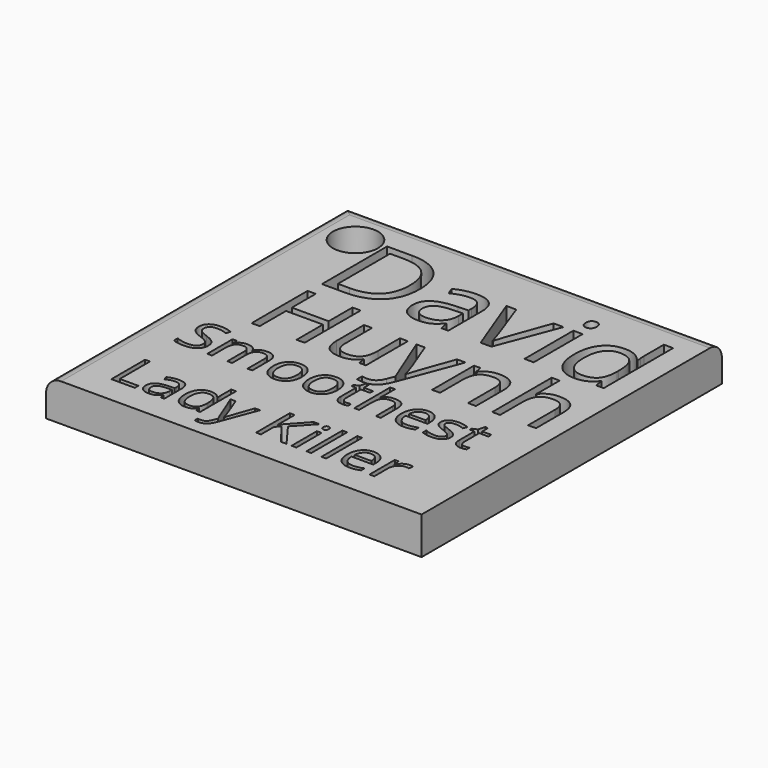
from build123d import *

# Parameters (mm, degrees)
F0_W         = 50
F0_H         = 50
F0_R         = 3
F1_DEPTH     = 5
F2_TEXT_SIZE = 13.0405990525
F4_DEPTH     = 5.001
F5_R         = 2
F6_TEXT_SIZE = 15.2046088971
F7_DEPTH     = 5.0010001
F3_TEXT_SIZE = 7.860235193
F8_DEPTH     = 5.0010001


# Not quite as in the source:
# - Text() gives the source's letters only with a copy of the font that has no kerning and outlines rounded to 1/6400 em; it was checked with that copy


with BuildPart() as f1:
    # F0 (on Top) → F1 (new body)
    with BuildSketch(Plane.XY):
        with Locations((25, -25)):
            Rectangle(F0_W, F0_H)
        with Locations((6, -6)):
            Circle(F0_R, mode=Mode.SUBTRACT)
    extrude(amount=F1_DEPTH)

    # F2 (on face) → F4 (cut, through all)
    with BuildSketch(Plane.XY.offset(5)):
        with Locations((8, -27.3892313178)):
            Text('Huynh', F2_TEXT_SIZE, font='Open Sans', text_align=(TextAlign.LEFT, TextAlign.BOTTOM))
    extrude(amount=-F4_DEPTH, mode=Mode.SUBTRACT)

    # F5
    f5_edges = [f1.edges().sort_by_distance(p)[0] for p in [
        (0, -25, 5),
        (25, 0, 5),
    ]]
    fillet(f5_edges, radius=F5_R)

    # F6 (on face) → F7 (cut, through all)
    with BuildSketch(Plane.XY.offset(5)):
        with Locations((8, -15.9473184059)):
            Text('David', F6_TEXT_SIZE, font='Open Sans', text_align=(TextAlign.LEFT, TextAlign.BOTTOM))
    extrude(amount=-F7_DEPTH, mode=Mode.SUBTRACT)

    # F3 (on face) → F8 (cut, through all)
    with BuildSketch(Plane.XY.offset(5)):
        with Locations((5, -35.6593693389)):
            Text('Smoothest', F3_TEXT_SIZE, font='Open Sans', text_align=(TextAlign.LEFT, TextAlign.BOTTOM))
        with Locations((5, -46.3492892014)):
            Text('Lady Killer', F3_TEXT_SIZE, font='Open Sans', text_align=(TextAlign.LEFT, TextAlign.BOTTOM))
    extrude(amount=-F8_DEPTH, mode=Mode.SUBTRACT)


solid = f1.part
